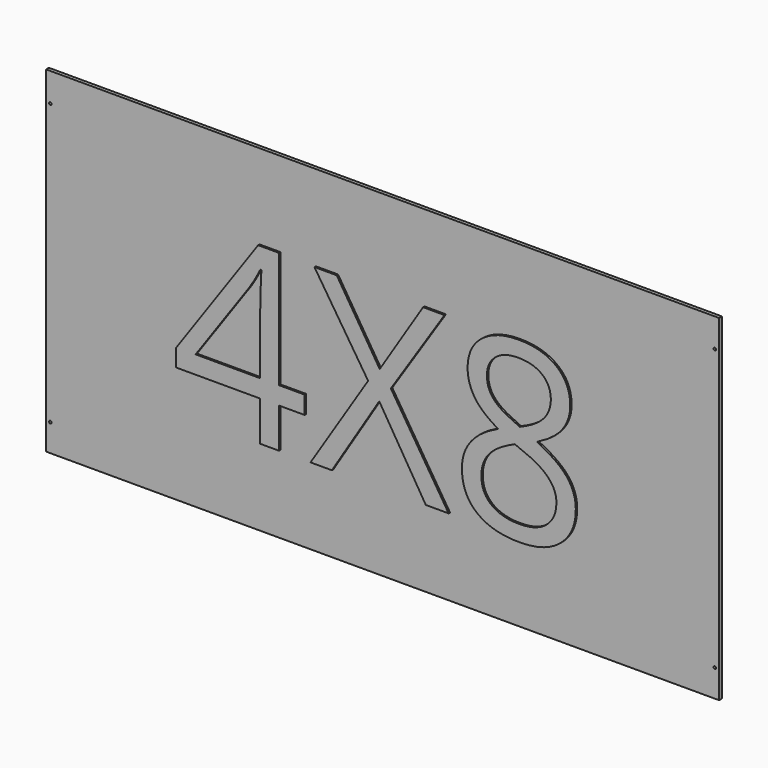
from build123d import *

# Parameters (mm, degrees)
F0_W         = 2438.4
F0_H         = 1219.2
F1_DEPTH     = 12.7
F2_R         = 4.7625
F3_DEPTH     = 12.701
F4_TEXT_SIZE = 879.0194664744
F5_DEPTH     = 6.35
F6_TEXT_SIZE = 879.0194664744
F7_DEPTH     = 6.35


# Not quite as in the source:
# - Text() gives the source's letters only with a copy of the font that has no kerning and outlines rounded to 1/6400 em; it was checked with that copy


with BuildPart() as f1:
    # F0 (on Front) → F1 (new body)
    with BuildSketch(Plane.XZ):
        with Locations((1219.2, 609.6)):
            Rectangle(F0_W, F0_H)
    extrude(amount=F1_DEPTH)

    # F2 (on face) → F3 (cut, through all)
    with BuildSketch(Plane.XZ.offset(12.7)):
        with Locations((2423.16, 1115.06)):
            Circle(F2_R)
        with Locations((2423.16, 99.06)):
            Circle(F2_R)
        with Locations((15.24, 99.06)):
            Circle(F2_R)
        with Locations((15.24, 1115.06)):
            Circle(F2_R)
    extrude(amount=-F3_DEPTH, mode=Mode.SUBTRACT)

    # F4 (on face) → F5 (join)
    with BuildSketch(Plane.XZ.offset(12.7)):
        with Locations((457.2, 281.5059841384)):
            Text('4X8', F4_TEXT_SIZE, font='Open Sans', text_align=(TextAlign.LEFT, TextAlign.BOTTOM))
    extrude(amount=F5_DEPTH)

    # F6 (on face) → F7 (join)
    with BuildSketch(Plane(origin=(0, 0, 0), x_dir=(-1, 0, 0), z_dir=(0, 1, 0))):
        with Locations((-1981.2, 281.5059841384)):
            Text('4X8', F6_TEXT_SIZE, font='Open Sans', text_align=(TextAlign.LEFT, TextAlign.BOTTOM))
    extrude(amount=F7_DEPTH)


solid = f1.part
